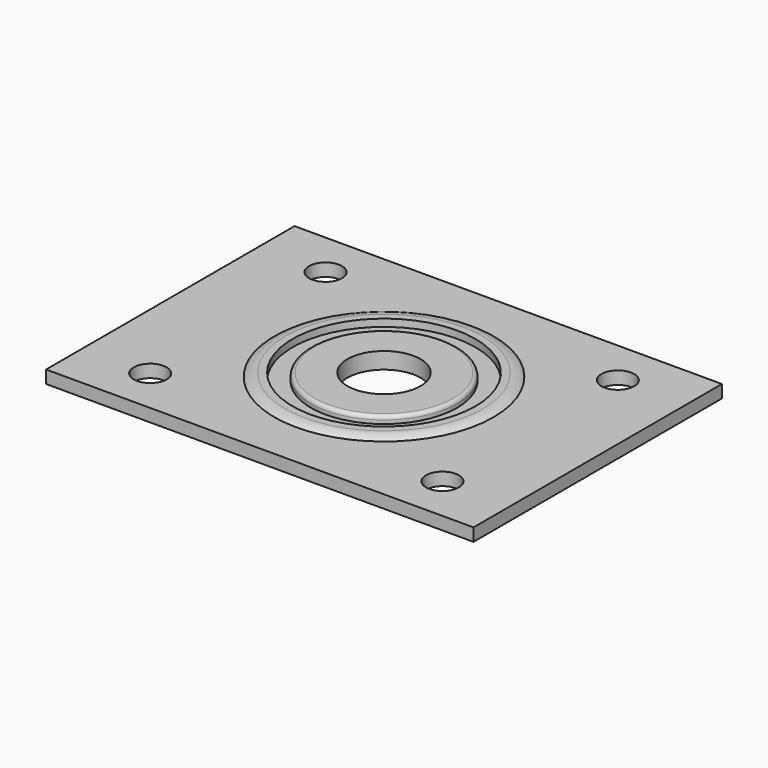
from build123d import *

# Parameters (mm, degrees)
F0_W      = 117
F0_H      = 85
F1_DEPTH  = 3.5
F2_R      = 4.5
F3_DEPTH  = 25
F4_R      = 30
F5_DEPTH  = 1
F7_R      = 25
F8_DEPTH  = 2
F9_R      = 20
F10_DEPTH = 2
F11_R     = 1
F12_R     = 10
F13_DEPTH = 25


# Not quite as in the source:
# - a fillet or chamfer that OpenCascade refuses, or shapes differently, is made with other operations: its cross-section is extruded or revolved along the edge and cut away or added


with BuildPart() as f1:
    # F0 (on Top) → F1 (new body)
    with BuildSketch(Plane.XY):
        Rectangle(F0_W, F0_H)
    extrude(amount=F1_DEPTH)

    # F2 (on face) → F3 (cut)
    with BuildSketch(Plane.XY.offset(3.5)):
        with Locations((40, 30)):
            Circle(F2_R)
        with Locations((-40, 30)):
            Circle(F2_R)
        with Locations((-40, -30)):
            Circle(F2_R)
        with Locations((40, -30)):
            Circle(F2_R)
    extrude(amount=-F3_DEPTH, mode=Mode.SUBTRACT)

    # F4 (on face) → F5 (join)
    with BuildSketch(Plane.XY.offset(3.5)):
        Circle(F4_R)
    extrude(amount=F5_DEPTH)

    # F6: fillet of radius 5 on 1 edges, made by hand

    # F6_s1 → F6_t2 (revolve, cut)
    with BuildSketch(Plane.XZ):
        with BuildLine():
            ThreePointArc((30, 3.5), (28.5811388301, 4.2434164903), (27, 4.5))
            Line((27, 4.5), (30, 4.5))
            Line((30, 4.5), (30, 3.5))
        make_face()
    revolve(axis=Axis((0, 0, 4.5), (0, 0, 1)), mode=Mode.SUBTRACT)

    # F7 (on face) → F8 (cut)
    with BuildSketch(Plane.XY.offset(4.5)):
        Circle(F7_R)
    extrude(amount=-F8_DEPTH, mode=Mode.SUBTRACT)

    # F9 (on face) → F10 (join)
    with BuildSketch(Plane.XY.offset(2.5)):
        Circle(F9_R)
    extrude(amount=F10_DEPTH)

    # F11
    f11_edges = [f1.edges().sort_by_distance(p)[0] for p in [
        (-20, 0, 4.5),
    ]]
    fillet(f11_edges, radius=F11_R)

    # F12 (on face) → F13 (cut)
    with BuildSketch(Plane.XY.offset(4.5)):
        Circle(F12_R)
    extrude(amount=-F13_DEPTH, mode=Mode.SUBTRACT)


solid = f1.part
